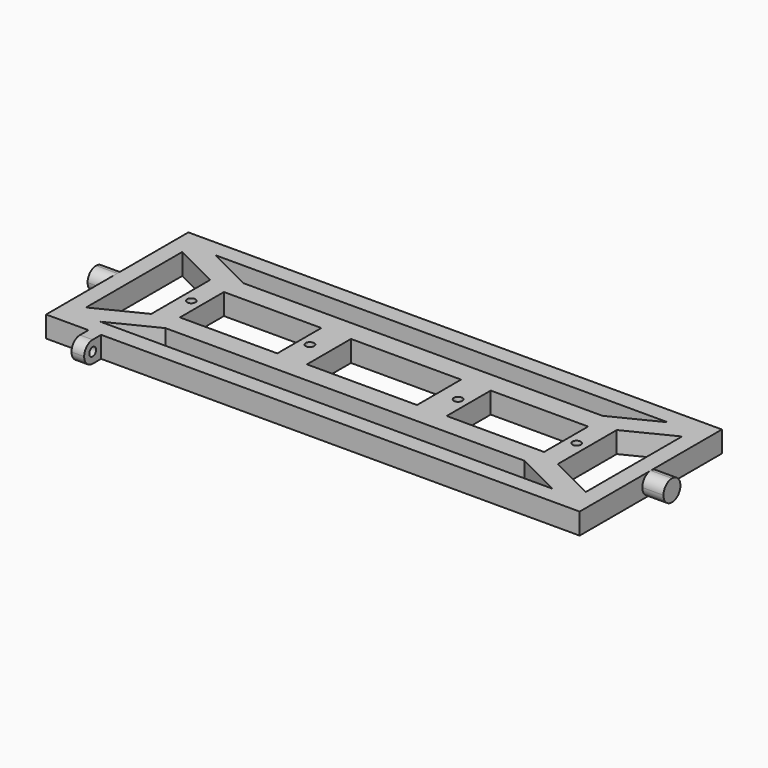
from build123d import *

# Parameters (mm, degrees)
F0_W     = 126
F0_H     = 42
F0_R     = 1
F0_W_2   = 23
F0_H_2   = 13
F0_W_3   = 26
F1_DEPTH = 5
F3_DEPTH = 5
F4_W     = 3
F4_H     = 5
F5_DEPTH = 5
F6_R     = 1
F7_DEPTH = 3


# Not quite as in the source:
# - a pattern or mirror of a feature is missing from the dataset's text; its kind, count and spacing are read off the source's solid


with BuildPart() as f1:
    # F0 (on Top) → F1 (new body)
    with BuildSketch(Plane.XY):
        Rectangle(F0_W, F0_H)
        Polygon((-7, -11.5), (7, -11.5), (42.4098300563, -11.5), (53.4098300563, -17), (-53.4098300563, -17), (-42.4098300563, -11.5), align=None, mode=Mode.SUBTRACT)
        Polygon((-59, 14.2049150281), (-48, 8.7049150281), (-48, -8.7049150281), (-59, -14.2049150281), align=None, mode=Mode.SUBTRACT)
        with Locations((-45.5, 0)):
            Circle(F0_R, mode=Mode.SUBTRACT)
        with Locations((-31.5, 0)):
            Rectangle(F0_W_2, F0_H_2, mode=Mode.SUBTRACT)
        with Locations((-17.5, 0)):
            Circle(F0_R, mode=Mode.SUBTRACT)
        Rectangle(F0_W_3, F0_H_2, mode=Mode.SUBTRACT)
        with Locations((17.5, 0)):
            Circle(F0_R, mode=Mode.SUBTRACT)
        with Locations((31.5, 0)):
            Rectangle(F0_W_2, F0_H_2, mode=Mode.SUBTRACT)
        with Locations((45.5, 0)):
            Circle(F0_R, mode=Mode.SUBTRACT)
        Polygon((48, -8.7049150281), (48, 8.7049150281), (59, 14.2049150281), (59, -14.2049150281), align=None, mode=Mode.SUBTRACT)
        Polygon((42.4098300563, 11.5), (7, 11.5), (-7, 11.5), (-42.4098300563, 11.5), (-53.4098300563, 17), (53.4098300563, 17), align=None, mode=Mode.SUBTRACT)
    extrude(amount=F1_DEPTH)

    # F2 (on face) → F3 (join)
    with BuildSketch(Plane(origin=(-63, 0, 0), x_dir=(0, -1, 0), z_dir=(-1, 0, 0))):
        with BuildLine():
            ThreePointArc((0, 0), (1.767766953, 0.732233047), (2.5, 2.5))
            ThreePointArc((2.5, 2.5), (1.7677669583, 4.2677669477), (1.5e-08, 5))
            ThreePointArc((1.5e-08, 5), (-2.5, 2.5000000075), (0, 0))
        make_face()
    f3 = extrude(amount=F3_DEPTH)

    # F3_copies: F3 across plane
    add(f3.mirror(Plane(origin=(0, 0, 0), x_dir=(0, 0, 1), z_dir=(1, 0, 0))))

    # F4 (on face) → F5 (join)
    with BuildSketch(Plane.XZ.offset(21)):
        with Locations((-51.5, 2.5)):
            Rectangle(F4_W, F4_H)
    extrude(amount=F5_DEPTH)

    # F6 (on face) → F7 (cut, through all)
    with BuildSketch(Plane(origin=(-53, 0, 0), x_dir=(0, -1, 0), z_dir=(-1, 0, 0))):
        with Locations((23.5, 2.5)):
            Circle(F6_R)
        with BuildLine():
            Line((26, 2.5), (26, 5))
            Line((26, 5), (23.5, 5))
            ThreePointArc((23.5, 5), (25.267766953, 4.267766953), (26, 2.5))
        make_face()
        with BuildLine():
            Line((26, 0), (26, 2.5))
            ThreePointArc((26, 2.5), (25.267766953, 0.732233047), (23.5, 0))
            Line((23.5, 0), (26, 0))
        make_face()
    extrude(amount=-F7_DEPTH, mode=Mode.SUBTRACT)


solid = f1.part
